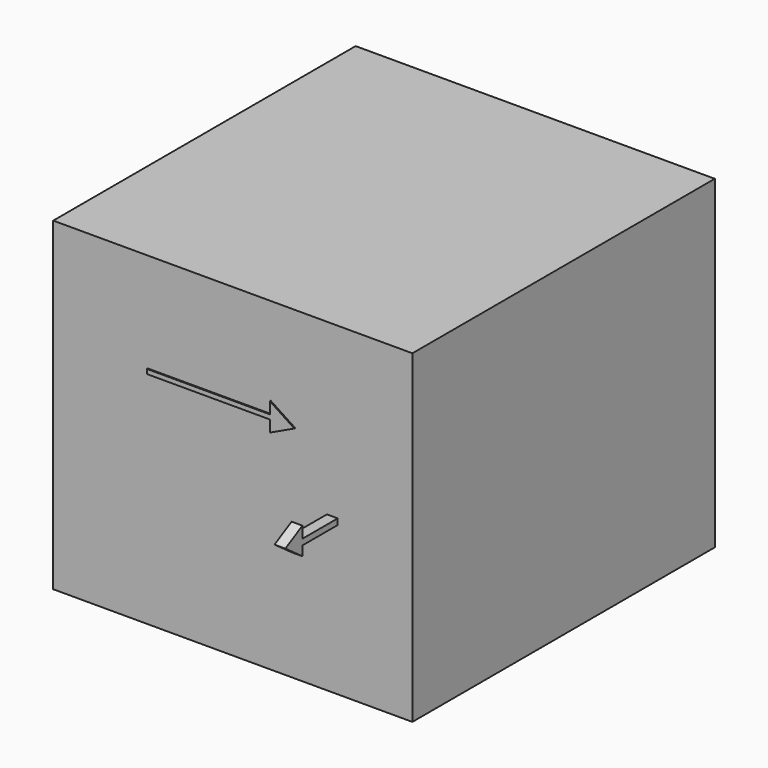
from build123d import *

# Parameters (mm, degrees)
F0_W     = 84.3321233988
F0_H     = 88.7495167553
F1_DEPTH = 76.2
F4_W     = 28.8745099679
F4_H     = 1.0582283139
F5_DEPTH = 0.254
F7_W     = 16.5562033653
F7_H     = 1.3796836138
F8_DEPTH = 2.54


# Not quite as in the source:
# - the program builds the solid bodies; features that only make, move or delete a surface that nothing else refers to are left out


with BuildPart() as f1:
    # F0 (on Top) → F1 (new body)
    with BuildSketch(Plane.XY):
        with Locations((4.1730180383, -8.0741699785)):
            Rectangle(F0_W, F0_H)
    extrude(amount=F1_DEPTH)

    # F4 (on face) → F5 (join)
    with BuildSketch(Plane.XZ.offset(52.4489283562)):
        with Locations((-1.3617197983, 52.3322783411)):
            Rectangle(F4_W, F4_H)
        Polygon((13.0755351856, 55.5825531483), (13.0755351856, 52.861392498), (13.0755351856, 51.8031641841), (13.0755351856, 49.0820072591), (18.8202019781, 51.8031641841), align=None)
    extrude(amount=F5_DEPTH)

    # F7 (on offset) → F8 (join)
    with BuildSketch(Plane(origin=(28.8089563389, 0, 0), x_dir=(0, -1, 0), z_dir=(-1, 0, 0))):
        with Locations((54.5372888446, 35.6855541468)):
            Rectangle(F7_W, F7_H)
        Polygon((62.8153905272, 39.0911102295), (62.8153905272, 36.3753959537), (62.8153905272, 34.9957123399), (62.8153905272, 32.7537246048), (67.8167492151, 36.3753959537), align=None)
    extrude(amount=F8_DEPTH)


solid = f1.part
